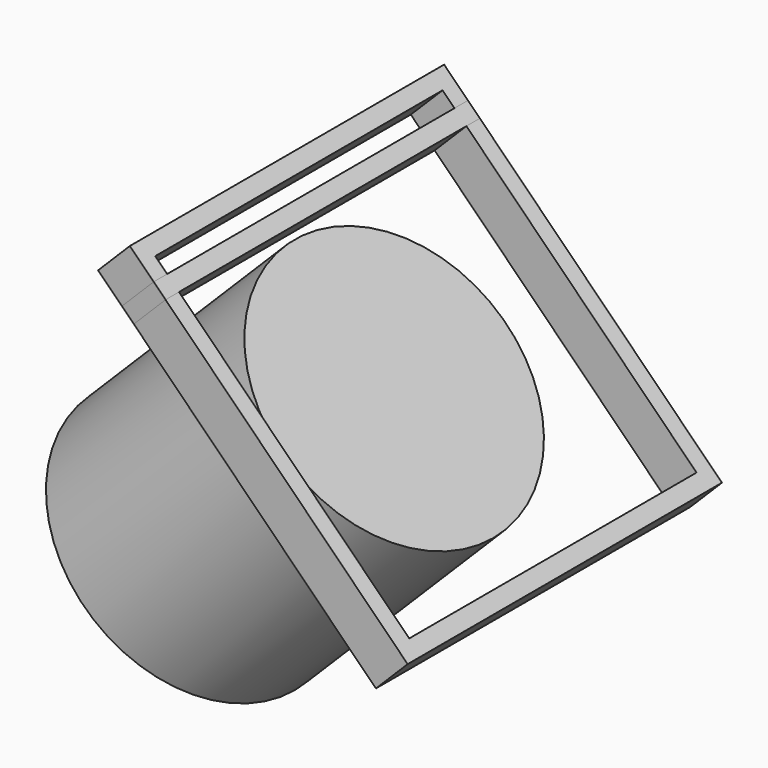
from build123d import *

# Parameters (mm, degrees)
F15_R     = 25
F16_DEPTH = 50
F15_W     = 3
F15_H     = 64
F15_H_2   = 3
F17_DEPTH = 8
F18_DEPTH = 8


with BuildPart() as f16:
    # F15 (on face) → F16 (new body)
    with BuildSketch(Plane(origin=(100.4091629285, 0, 100.4091629285), x_dir=(0.7071067812, 0, -0.7071067812), z_dir=(0.7071067812, 0, 0.7071067812))):
        with Locations((0, -35)):
            Circle(F15_R)
    extrude(amount=-F16_DEPTH)


with BuildPart() as f17:
    # F15 (on face) → F17 (new body)
    with BuildSketch(Plane(origin=(100.4091629285, 0, 100.4091629285), x_dir=(0.7071067812, 0, -0.7071067812), z_dir=(0.7071067812, 0, 0.7071067812))):
        with Locations((-27.5, -35)):
            Rectangle(F15_W, F15_H)
        with Locations((-27.5, -68.5)):
            Rectangle(F15_W, F15_H_2)
        with Locations((-27.5, -1.5)):
            Rectangle(F15_W, F15_H_2)
    extrude(amount=F17_DEPTH)


with BuildPart() as f18:
    # F15 (on face) → F18 (new body)
    with BuildSketch(Plane(origin=(100.4091629285, 0, 100.4091629285), x_dir=(0.7071067812, 0, -0.7071067812), z_dir=(0.7071067812, 0, 0.7071067812))):
        Polygon((-35, 0), (-35, -70), (-29, -70), (-29, -67), (-32, -67), (-32, -3), (-29, -3), (-29, 0), align=None)
    extrude(amount=F18_DEPTH)


with BuildPart() as f18b:
    # F15 (on face) → F18, piece 2 (new body)
    with BuildSketch(Plane(origin=(100.4091629285, 0, 100.4091629285), x_dir=(0.7071067812, 0, -0.7071067812), z_dir=(0.7071067812, 0, 0.7071067812))):
        Polygon((-26, -67), (-26, -70), (35, -70), (35, 0), (-26, 0), (-26, -3), (0, -3), (32, -3), (32, -67), (0, -67), align=None)
    extrude(amount=F18_DEPTH)


solid = Compound([f16.part, f17.part, f18.part, f18b.part])
